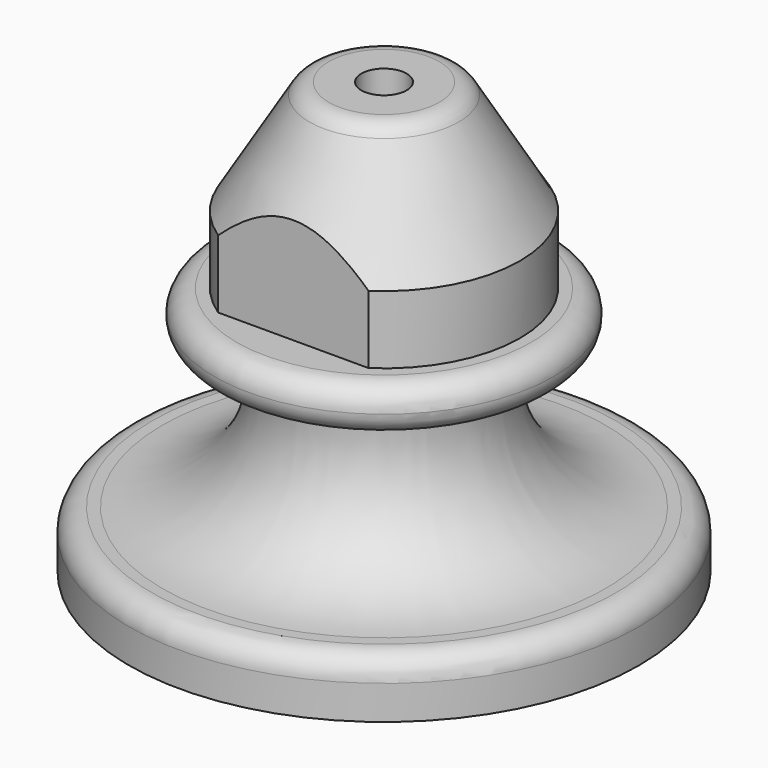
from build123d import *

# Parameters (mm, degrees)
F2_R     = 1.99999
F4_DEPTH = 16


# Not quite as in the source:
# - a fillet or chamfer is up to 0.001 mm smaller than in the source, because OpenCascade refuses the exact size


with BuildPart() as f1:
    # F0 (on Front) → F1 (revolve)
    with BuildSketch(Plane.XZ):
        with BuildLine():
            Line((-2, 22.5393301398), (-2, 35.5393301398))
            Line((-2, 35.5393301398), (-6, 35.5393301398))
            Line((-6, 35.5393301398), (-12, 25.5393301398))
            Line((-12, 25.5393301398), (-12, 19.5393301398))
            Line((-12, 19.5393301398), (-15, 19.5393301398))
            Line((-15, 19.5393301398), (-15, 15.5393301398))
            Line((-15, 15.5393301398), (-10, 15.5393301398))
            ThreePointArc((-10, 15.5393301398), (-11.4771342659, 6.6232503567), (-19.5393920142, 2.5393301398))
            Line((-19.5393920142, 2.5393301398), (-22.5, 2.5393301398))
            Line((-22.5, 2.5393301398), (-22.5, -2.4606698602))
            Line((-22.5, -2.4606698602), (-19.5, -2.4606698602))
            Line((-19.5, -2.4606698602), (-19.5, 0))
            ThreePointArc((-19.5, 0), (-10.6587866296, 3.6865791499), (-7, 12.5393301398))
            Line((-7, 12.5393301398), (-7, 22.5393301398))
            Line((-7, 22.5393301398), (-2, 22.5393301398))
        make_face()
    revolve(axis=Axis((0, 0, 14.2342122272), (0, 0, -1)))

    # F2 (radius 2 in the source; OpenCascade refuses exactly that, so slightly less here)
    f2_edges = [f1.edges().sort_by_distance(p)[0] for p in [
        (22.5, 0, 2.53933),
        (15, 0, 15.53933),
        (15, 0, 19.53933),
        (6, 0, 35.53933),
        (19.5, 0, 0),
        (7, 0, 12.53933),
        (-10.658787, 0, 3.686579),
        (7, 0, 22.53933),
        (10, 0, 15.53933),
    ]]
    fillet(f2_edges, radius=F2_R)

    # F3 (on face) → F4 (cut, through all)
    with BuildSketch(Plane.XY.offset(35.5393301398)):
        with BuildLine():
            Line((-8.3066238629, 10), (8.3066238629, 10))
            ThreePointArc((8.3066238629, 10), (0, 13), (-8.3066238629, 10))
        make_face()
        with BuildLine():
            ThreePointArc((-8.3066238629, -10), (0, -13), (8.3066238629, -10))
            Line((8.3066238629, -10), (-8.3066238629, -10))
        make_face()
    extrude(amount=-F4_DEPTH, mode=Mode.SUBTRACT)


solid = f1.part
